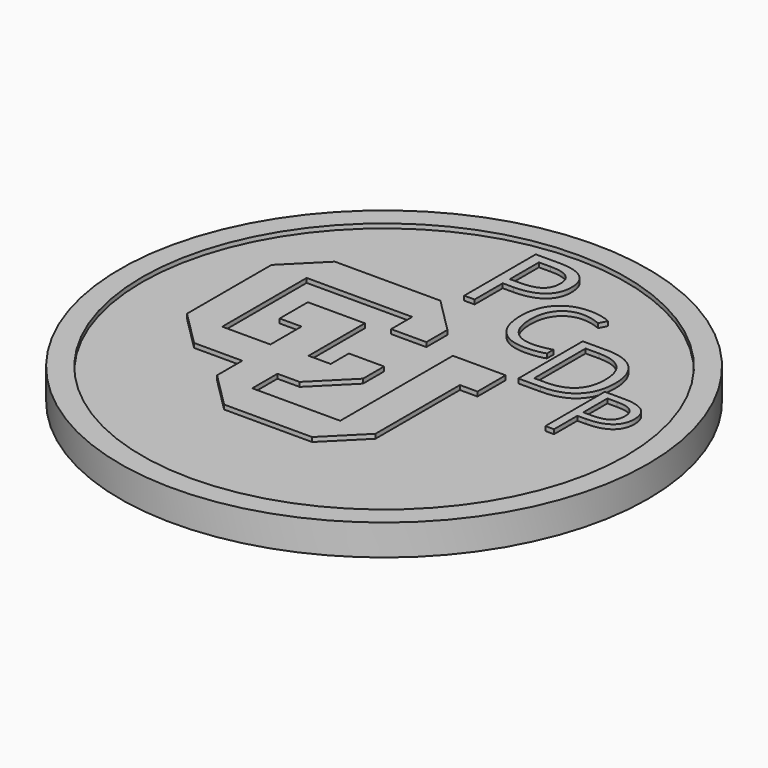
from build123d import *

# Parameters (mm, degrees)
F0_R           = 38.1
F1_DEPTH       = 3.81
F2_R           = 38.1
F2_R_2         = 34.925
F2_TEXT_SIZE   = 16.2687993401
F2_TEXT_SIZE_2 = 18.0764434238
F2_TEXT_SIZE_3 = 15.003449193
F2_TEXT_SIZE_4 = 15.7265070205
F3_DEPTH       = 0.635
F4_TEXT_SIZE   = 19.4162317914
F4_TEXT_SIZE_2 = 18.3375507024
F5_DEPTH       = 0.635


# Not quite as in the source:
# - Text() gives the source's letters only with a copy of the font that has no kerning and outlines rounded to 1/6400 em; it was checked with that copy


with BuildPart() as f1:
    # F0 (on Top) → F1 (new body)
    with BuildSketch(Plane.XY):
        Circle(F0_R)
    extrude(amount=F1_DEPTH)

    # F2 (on face) → F3 (join)
    with BuildSketch(Plane.XY.offset(3.81)):
        Circle(F2_R)
        Circle(F2_R_2, mode=Mode.SUBTRACT)
        Polygon((0, -3.81), (0, 0), (-5.08, 0), (-5.08, -3.2792999409), (-8.2786227894, -3.2792999409), (-8.2786227894, 6.8807000591), (-16.51, 6.8807000591), (-16.51, 1.8007000591), (-13.3586227894, 1.8007000591), (-13.3586227894, -3.81), (-20.32, -3.81), (-20.32, 11.43), (-5.08, 11.43), (-5.08, 7.62), (0, 7.62), (0, 11.43), (-5.08, 16.51), (-20.32, 16.51), (-25.4, 11.43), (-25.4, -3.81), (-20.32, -8.89), (-13.3586227894, -8.89), (-13.3586227894, -13.4392999409), (-8.2786227894, -18.5192999409), (4.4213772106, -18.5192999409), (9.5013772106, -13.4392999409), (9.5013772106, 1.8007000591), (12.0413772106, 1.8007000591), (12.0413772106, 6.8807000591), (4.4213772106, 6.8807000591), (4.4213772106, -13.4392999409), (-8.2786227894, -13.4392999409), (-8.2786227894, -8.89), (-5.08, -8.89), align=None)
        with Locations((12.049453333, 7.1704220027)):
            Text('D', F2_TEXT_SIZE, font='Open Sans', text_align=(TextAlign.LEFT, TextAlign.BOTTOM))
        with Locations((-5.5208513513, 19.1442575306)):
            Text('P', F2_TEXT_SIZE_2, font='Open Sans', text_align=(TextAlign.LEFT, TextAlign.BOTTOM))
        with Locations((21.8107327819, 0)):
            Text('P', F2_TEXT_SIZE_3, font='Open Sans', text_align=(TextAlign.LEFT, TextAlign.BOTTOM))
        with Locations((3.3293755259, 13.6779453605)):
            Text('C', F2_TEXT_SIZE_4, font='Open Sans', text_align=(TextAlign.LEFT, TextAlign.BOTTOM))
    extrude(amount=F3_DEPTH)

    # F4 (on face) → F5 (join)
    with BuildSketch(Plane(origin=(0, 0, 0), x_dir=(1, 0, 0), z_dir=(0, 0, -1))):
        with Locations((-29.6292807907, 1.9543780945)):
            Text('Alyssa', F4_TEXT_SIZE, font='Arimo', text_align=(TextAlign.LEFT, TextAlign.BOTTOM))
        with Locations((-27.6876576245, -16.4910405874)):
            Text('Gasca', F4_TEXT_SIZE_2, font='Open Sans', text_align=(TextAlign.LEFT, TextAlign.BOTTOM))
    extrude(amount=F5_DEPTH)


solid = f1.part
